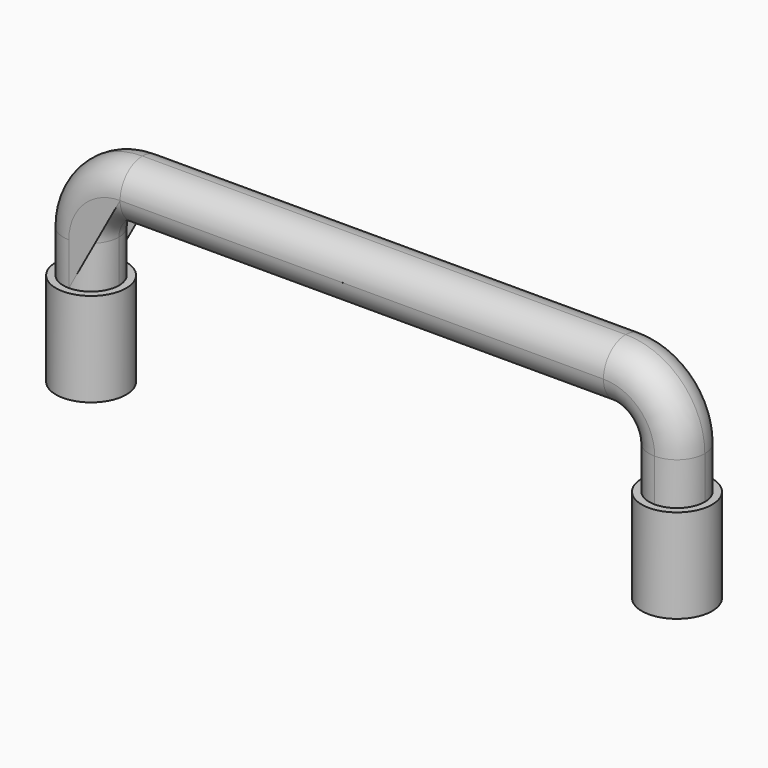
from build123d import *

# Parameters (mm, degrees)
F1_DEPTH = 60.325
F2_R     = 30.16249
F3_R     = 38.1
F3_R_2   = 30.1625
F4_DEPTH = 50.8
F5_R     = 38.1
F5_R_2   = 30.1625
F6_DEPTH = 50.8


# Not quite as in the source:
# - a fillet or chamfer is up to 0.001 mm smaller than in the source, because OpenCascade refuses the exact size


with BuildPart() as f1:
    # F0 (on Front) → F1 (new body)
    with BuildSketch(Plane.XZ):
        with BuildLine():
            Line((-347.6625, 0), (-317.5, 0))
            Line((-317.5, 0), (-287.3375, 0))
            Line((-287.3375, 0), (-287.3375, 96.8375))
            ThreePointArc((-287.3375, 96.8375), (-279.8980122421, 114.7980122421), (-261.9375, 122.2375))
            Line((-261.9375, 122.2375), (261.9375, 122.2375))
            ThreePointArc((261.9375, 122.2375), (279.8980122421, 114.7980122421), (287.3375, 96.8375))
            Line((287.3375, 96.8375), (287.3375, 0))
            Line((287.3375, 0), (317.5, 0))
            Line((317.5, 0), (347.6625, 0))
            Line((347.6625, 0), (347.6625, 96.8375))
            ThreePointArc((347.6625, 96.8375), (322.5542288172, 157.4542288172), (261.9375, 182.5625))
            Line((261.9375, 182.5625), (-261.9375, 182.5625))
            ThreePointArc((-261.9375, 182.5625), (-322.5542288172, 157.4542288172), (-347.6625, 96.8375))
            Line((-347.6625, 96.8375), (-347.6625, 0))
        make_face()
    extrude(amount=F1_DEPTH)

    # F2 (radius 30.1625 in the source; OpenCascade refuses exactly that, so slightly less here)
    f2_edges = [f1.edges().sort_by_distance(p)[0] for p in [
        (0, -60.325, 182.5625),
        (0, -60.325, 122.2375),
        (0, 0, 182.5625),
        (0, 0, 122.2375),
    ]]
    fillet(f2_edges, radius=F2_R)

    # F3 (on face) → F4 (join, symmetric)
    with BuildSketch(Plane(origin=(0, 0, 0), x_dir=(1, 0, 0), z_dir=(0, 0, -1))):
        with Locations((-317.5, 30.1625)):
            Circle(F3_R)
        with Locations((-317.5, 30.1625)):
            Circle(F3_R_2, mode=Mode.SUBTRACT)
    extrude(amount=F4_DEPTH, both=True)

    # F5 (on face) → F6 (join, symmetric)
    with BuildSketch(Plane(origin=(0, 0, 0), x_dir=(1, 0, 0), z_dir=(0, 0, -1))):
        with Locations((317.5, 30.1625)):
            Circle(F5_R)
        with Locations((317.5, 30.1625)):
            Circle(F5_R_2, mode=Mode.SUBTRACT)
    extrude(amount=F6_DEPTH, both=True)


solid = f1.part
